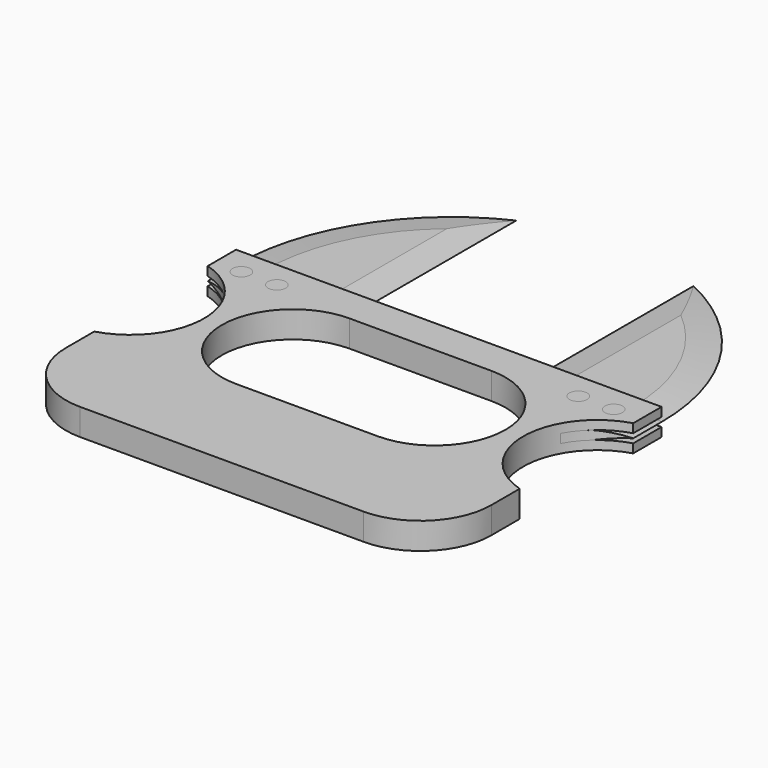
from build123d import *

# Parameters (mm, degrees)
F1_DEPTH      = 2.38125
F1_DEPTH_BACK = 2.38125
F3_DEPTH      = 0.79375
F3_DEPTH_BACK = 0.79375
F4_DEPTH      = 0.79375
F4_DEPTH_BACK = 0.79375
F5_R          = 1.5875
F6_DEPTH      = 2.38125
F6_DEPTH_BACK = 2.38125
F7_DEPTH      = 2.38125
F7_DEPTH_BACK = 2.38125
F8_T1_DEPTH   = 61.3292860819
F8_T3_DEPTH   = 19.552143041
F8_T6_ANGLE   = 84.5666435794
F8_2_T1_DEPTH = 61.3292860819
F8_2_T3_DEPTH = 19.552143041
F8_2_T6_ANGLE = 84.5666435794
F9_T1_DEPTH   = 61.3292860819
F9_T3_DEPTH   = 19.552143041
F9_T6_ANGLE   = 84.5666435794
F9_2_T1_DEPTH = 61.3292860819
F9_2_T3_DEPTH = 19.552143041
F9_2_T6_ANGLE = 84.5666435794


# Not quite as in the source:
# - a fillet or chamfer that OpenCascade refuses, or shapes differently, is made with other operations: its cross-section is extruded or revolved along the edge and cut away or added


with BuildPart() as f1:
    # F0 (on Top) → F1 (new body, two sides)
    with BuildSketch(Plane.XY) as f1_sk:
        with BuildLine():
            Line((-25.4, -25.4), (25.4, -25.4))
            ThreePointArc((25.4, -25.4), (34.3802561211, -21.6802561211), (38.1, -12.7))
            Line((38.1, -12.7), (38.1, -6.35))
            ThreePointArc((38.1, -6.35), (28.575, 6.35), (38.1, 19.05))
            Line((38.1, 19.05), (38.1, 25.4))
            Line((38.1, 25.4), (-38.1, 25.4))
            Line((-38.1, 25.4), (-38.1, 19.05))
            ThreePointArc((-38.1, 19.05), (-28.575, 6.35), (-38.1, -6.35))
            Line((-38.1, -6.35), (-38.1, -12.7))
            ThreePointArc((-38.1, -12.7), (-34.3802561211, -21.6802561211), (-25.4, -25.4))
        make_face()
        with BuildLine():
            Line((12.7, -6.35), (-12.7, -6.35))
            ThreePointArc((-12.7, -6.35), (-25.4, 6.35), (-12.7, 19.05))
            Line((-12.7, 19.05), (12.7, 19.05))
            ThreePointArc((12.7, 19.05), (25.4, 6.35), (12.7, -6.35))
        make_face(mode=Mode.SUBTRACT)
    extrude(amount=F1_DEPTH)
    extrude(f1_sk.sketch, amount=-F1_DEPTH_BACK)

    # F2 (on Top) → F3 (cut, two sides)
    with BuildSketch(Plane.XY) as f3_sk:
        with BuildLine():
            ThreePointArc((-15.875, 60.325), (-32.0725920002, 46.0984676365), (-38.1, 25.4))
            Line((-38.1, 25.4), (-38.1, 19.05))
            ThreePointArc((-38.1, 19.05), (-33.5169876558, 16.661814328), (-30.1986356278, 12.7))
            Line((-30.1986356278, 12.7), (-15.875, 25.4))
            Line((-15.875, 25.4), (-15.875, 60.325))
        make_face()
        with BuildLine():
            Line((15.875, 60.325), (15.875, 25.4))
            Line((15.875, 25.4), (30.1986356278, 12.7))
            ThreePointArc((30.1986356278, 12.7), (33.5169876558, 16.661814328), (38.1, 19.05))
            Line((38.1, 19.05), (38.1, 25.4))
            ThreePointArc((38.1, 25.4), (32.0725920002, 46.0984676365), (15.875, 60.325))
        make_face()
    extrude(amount=F3_DEPTH, mode=Mode.SUBTRACT)
    extrude(f3_sk.sketch, amount=-F3_DEPTH_BACK, mode=Mode.SUBTRACT)


with BuildPart() as f4:
    # F2 (on Top) → F4 (new body, two sides)
    with BuildSketch(Plane.XY) as f4_sk:
        with BuildLine():
            Line((15.875, 60.325), (15.875, 25.4))
            Line((15.875, 25.4), (30.1986356278, 12.7))
            ThreePointArc((30.1986356278, 12.7), (33.5169876558, 16.661814328), (38.1, 19.05))
            Line((38.1, 19.05), (38.1, 25.4))
            ThreePointArc((38.1, 25.4), (32.0725920002, 46.0984676365), (15.875, 60.325))
        make_face()
    extrude(amount=F4_DEPTH)
    extrude(f4_sk.sketch, amount=-F4_DEPTH_BACK)


with BuildPart() as f4b:
    # F2 (on Top) → F4, piece 2 (new body, two sides)
    with BuildSketch(Plane.XY) as f4_2_sk:
        with BuildLine():
            ThreePointArc((-15.875, 60.325), (-32.0725920002, 46.0984676365), (-38.1, 25.4))
            Line((-38.1, 25.4), (-38.1, 19.05))
            ThreePointArc((-38.1, 19.05), (-33.5169876558, 16.661814328), (-30.1986356278, 12.7))
            Line((-30.1986356278, 12.7), (-15.875, 25.4))
            Line((-15.875, 25.4), (-15.875, 60.325))
        make_face()
    extrude(amount=F4_DEPTH)
    extrude(f4_2_sk.sketch, amount=-F4_DEPTH_BACK)


with BuildPart() as f6_tool:
    # F5 (on Top) → F6 (new body, two sides)
    with BuildSketch(Plane.XY) as f6_sk:
        with Locations((-26.9875, 20.6375)):
            Circle(F5_R)
        with Locations((26.9875, 20.6375)):
            Circle(F5_R)
        with Locations((-33.3375, 20.6375)):
            Circle(F5_R)
        with Locations((33.3375, 20.6375)):
            Circle(F5_R)
    extrude(amount=F6_DEPTH)
    extrude(f6_sk.sketch, amount=-F6_DEPTH_BACK)


with BuildPart() as f1_1:
    add(f1.part)

    # F6: cut by f6_tool
    add(f6_tool.part, mode=Mode.SUBTRACT)


with BuildPart() as f4_1:
    add(f4.part)

    # F6: cut by f6_tool
    add(f6_tool.part, mode=Mode.SUBTRACT)

    # F8: chamfer of 0.79375 x 5.08 on 2 edges, made by hand

    # F8_s2 → F8_t1 (cut)
    with BuildSketch(Plane.XZ.offset(-73.527143041)):
        Polygon((15.875, 0), (20.955, 0.79375), (15.875, 0.79375), align=None)
    extrude(amount=F8_T1_DEPTH, mode=Mode.SUBTRACT)

    # F8_s4 → F8_t3 (cut)
    with BuildSketch(Plane.XZ.offset(-25.4)):
        Polygon((33.02, 0.79375), (38.1, 0), (38.1, 0.79375), align=None)
    extrude(amount=F8_T3_DEPTH, mode=Mode.SUBTRACT)

    # F8_s5 → F8_t6 (revolve, cut)
    with BuildSketch(Plane.XZ.offset(-25.4)):
        Polygon((38.1, 0), (33.02, 0.79375), (38.1, 0.79375), align=None)
    revolve(axis=Axis((-0.4535714286, 25.4, 0.79375), (0, 0, 1)), revolution_arc=F8_T6_ANGLE, mode=Mode.SUBTRACT)

    # F9: chamfer of 0.79375 x 5.08 on 2 edges, made by hand

    # F9_s2 → F9_t1 (cut)
    with BuildSketch(Plane.XZ.offset(-73.527143041)):
        Polygon((15.875, 0), (20.955, -0.79375), (15.875, -0.79375), align=None)
    extrude(amount=F9_T1_DEPTH, mode=Mode.SUBTRACT)

    # F9_s4 → F9_t3 (cut)
    with BuildSketch(Plane.XZ.offset(-25.4)):
        Polygon((33.02, -0.79375), (38.1, 0), (38.1, -0.79375), align=None)
    extrude(amount=F9_T3_DEPTH, mode=Mode.SUBTRACT)

    # F9_s5 → F9_t6 (revolve, cut)
    with BuildSketch(Plane.XZ.offset(-25.4)):
        Polygon((38.1, 0), (33.02, -0.79375), (38.1, -0.79375), align=None)
    revolve(axis=Axis((-0.4535714286, 25.4, -0.79375), (0, 0, 1)), revolution_arc=F9_T6_ANGLE, mode=Mode.SUBTRACT)


with BuildPart() as f4b_1:
    add(f4b.part)

    # F6: cut by f6_tool
    add(f6_tool.part, mode=Mode.SUBTRACT)

    # F8#2: chamfer of 0.79375 x 5.08 on 2 edges, made by hand

    # F8_2_s2 → F8_2_t1 (cut)
    with BuildSketch(Plane.XZ.offset(-73.527143041)):
        Polygon((-20.955, 0.79375), (-15.875, 0), (-15.875, 0.79375), align=None)
    extrude(amount=F8_2_T1_DEPTH, mode=Mode.SUBTRACT)

    # F8_2_s4 → F8_2_t3 (cut)
    with BuildSketch(Plane.XZ.offset(-25.4)):
        Polygon((-33.02, 0.79375), (-38.1, 0), (-38.1, 0.79375), align=None)
    extrude(amount=F8_2_T3_DEPTH, mode=Mode.SUBTRACT)

    # F8_2_s5 → F8_2_t6 (revolve, cut)
    with BuildSketch(Plane(origin=(2.8437713092, 0.2704860048, 0), x_dir=(0, 0, 1), z_dir=(0.995507008, 0.094687893, 0))):
        Polygon((0.79375, -58.7165017082), (0, -63.7965017082), (0.79375, -63.7965017082), align=None)
    revolve(axis=Axis((0.4535714286, 25.4, 0.79375), (0, 0, 1)), revolution_arc=F8_2_T6_ANGLE, mode=Mode.SUBTRACT)

    # F9#2: chamfer of 0.79375 x 5.08 on 2 edges, made by hand

    # F9_2_s2 → F9_2_t1 (cut)
    with BuildSketch(Plane.XZ.offset(-73.527143041)):
        Polygon((-20.955, -0.79375), (-15.875, 0), (-15.875, -0.79375), align=None)
    extrude(amount=F9_2_T1_DEPTH, mode=Mode.SUBTRACT)

    # F9_2_s4 → F9_2_t3 (cut)
    with BuildSketch(Plane.XZ.offset(-25.4)):
        Polygon((-33.02, -0.79375), (-38.1, 0), (-38.1, -0.79375), align=None)
    extrude(amount=F9_2_T3_DEPTH, mode=Mode.SUBTRACT)

    # F9_2_s5 → F9_2_t6 (revolve, cut)
    with BuildSketch(Plane(origin=(2.8437713092, 0.2704860048, 0), x_dir=(0, 0, 1), z_dir=(0.995507008, 0.094687893, 0))):
        Polygon((-0.79375, -58.7165017082), (0, -63.7965017082), (-0.79375, -63.7965017082), align=None)
    revolve(axis=Axis((0.4535714286, 25.4, -0.79375), (0, 0, 1)), revolution_arc=F9_2_T6_ANGLE, mode=Mode.SUBTRACT)


with BuildPart() as f7:
    # F5 (on Top) → F7 (new body, two sides)
    with BuildSketch(Plane.XY) as f7_sk:
        with Locations((-33.3375, 20.6375)):
            Circle(F5_R)
    extrude(amount=F7_DEPTH)
    extrude(f7_sk.sketch, amount=-F7_DEPTH_BACK)


with BuildPart() as f7b:
    # F5 (on Top) → F7, piece 2 (new body, two sides)
    with BuildSketch(Plane.XY) as f7_2_sk:
        with Locations((-26.9875, 20.6375)):
            Circle(F5_R)
    extrude(amount=F7_DEPTH)
    extrude(f7_2_sk.sketch, amount=-F7_DEPTH_BACK)


with BuildPart() as f7c:
    # F5 (on Top) → F7, piece 3 (new body, two sides)
    with BuildSketch(Plane.XY) as f7_3_sk:
        with Locations((26.9875, 20.6375)):
            Circle(F5_R)
    extrude(amount=F7_DEPTH)
    extrude(f7_3_sk.sketch, amount=-F7_DEPTH_BACK)


with BuildPart() as f7d:
    # F5 (on Top) → F7, piece 4 (new body, two sides)
    with BuildSketch(Plane.XY) as f7_4_sk:
        with Locations((33.3375, 20.6375)):
            Circle(F5_R)
    extrude(amount=F7_DEPTH)
    extrude(f7_4_sk.sketch, amount=-F7_DEPTH_BACK)


solid = Compound([f1_1.part, f4_1.part, f4b_1.part, f7.part, f7b.part, f7c.part, f7d.part])
